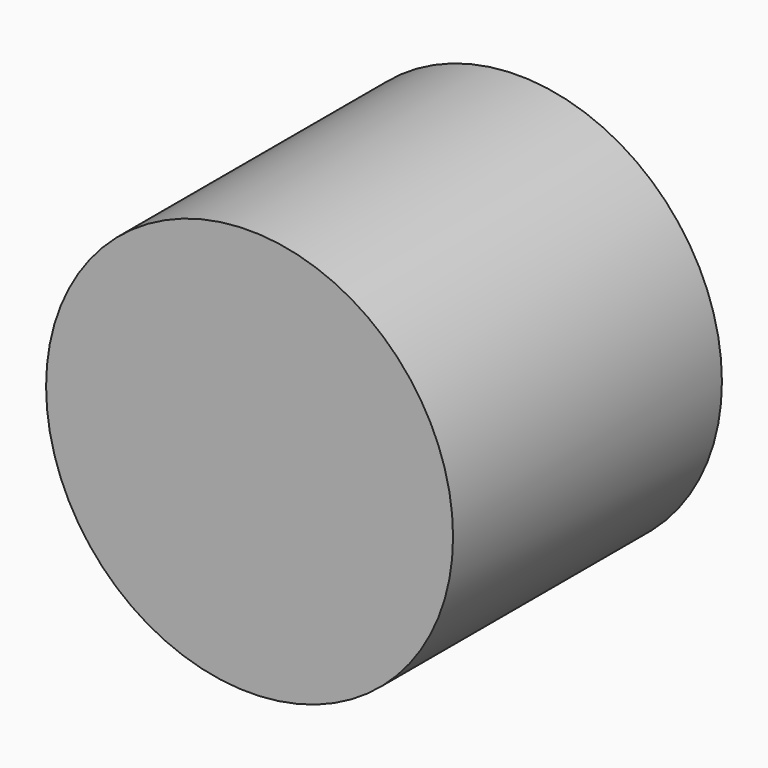
from build123d import *

# Parameters (mm, degrees)
F0_R     = 15.378921852
F1_DEPTH = 25.4


# Not quite as in the source:
# - an extrude whose draft closes it to a point is written as a loft to that point


with BuildPart() as f1:
    # F0 (on Front) → F1 (new body)
    with BuildSketch(Plane.XZ):
        Circle(F0_R)
    extrude(amount=F1_DEPTH)

    # F0 (on Front) → F2 section 0
    with BuildSketch(Plane.XZ, mode=Mode.PRIVATE) as f2_s0:
        Circle(F0_R)
    loft([f2_s0.sketch, Vertex(0, -1.3454813193, 0)], ruled=True, mode=Mode.SUBTRACT)


solid = f1.part
